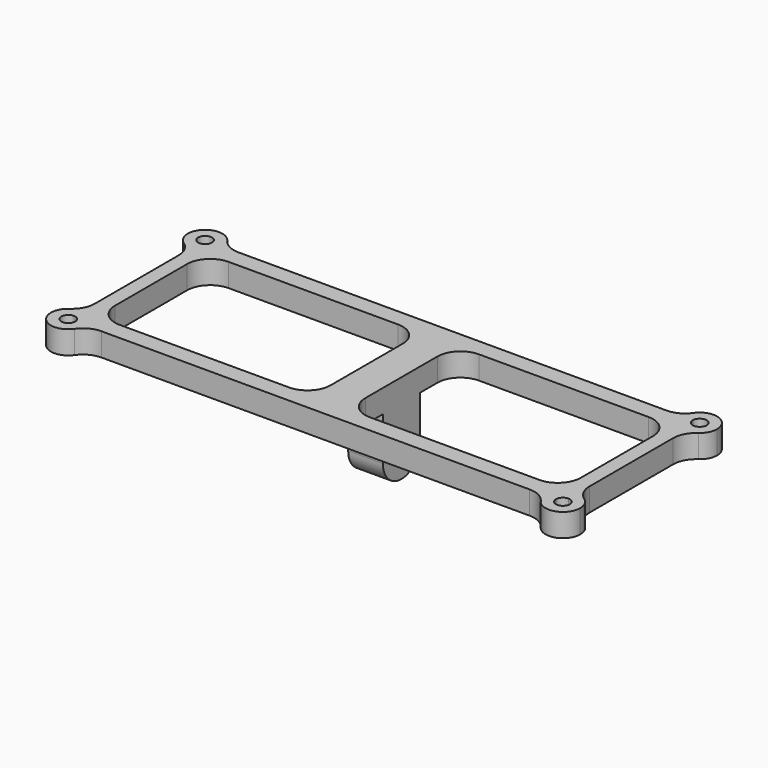
from build123d import *

# Parameters (mm, degrees)
F0_W     = 3
F0_H     = 0.7113954189
F0_H_2   = 11.7951147258
F1_DEPTH = 2
F2_R     = 2
F3_W     = 4
F3_H     = 7.7592988014
F3_R     = 0.75
F4_DEPTH = 3
F5_R     = 1.99999


# Not quite as in the source:
# - a fillet or chamfer is up to 0.001 mm smaller than in the source, because OpenCascade refuses the exact size


with BuildPart() as f1:
    # F0 (on Top) → F1 (new body)
    with BuildSketch(Plane.XY):
        with BuildLine():
            ThreePointArc((-21.4, 5.9), (-20.3393398282, 6.3393398282), (-19.9, 7.4))
            Line((-19.9, 7.4), (-20.8, 7.4))
            ThreePointArc((-20.8, 7.4), (-20.9757359313, 6.9757359313), (-21.4, 6.8))
            Line((-21.4, 6.8), (-21.4, 5.9))
        make_face()
        with BuildLine():
            Line((-20.8, 7.4), (-19.9, 7.4))
            ThreePointArc((-19.9, 7.4), (-22.4606601718, 8.4606601718), (-21.4, 5.9))
            Line((-21.4, 5.9), (-21.4, 6.8))
            ThreePointArc((-21.4, 6.8), (-21.8242640687, 7.8242640687), (-20.8, 7.4))
        make_face()
        with BuildLine():
            Line((19.9, 7.4), (-19.9, 7.4))
            ThreePointArc((-19.9, 7.4), (-20.3393398282, 6.3393398282), (-21.4, 5.9))
            Line((-21.4, 5.9), (-21.4, -5.9))
            ThreePointArc((-21.4, -5.9), (-20.3393398282, -6.3393398282), (-19.9, -7.4))
            Line((-19.9, -7.4), (19.9, -7.4))
            ThreePointArc((19.9, -7.4), (20.0395252165, -6.7682497618), (20.4321444846, -6.2540263086))
            Line((20.4321444846, -6.2540263086), (20.4321444846, 6.2540263086))
            ThreePointArc((20.4321444846, 6.2540263086), (20.0395252165, 6.7682497618), (19.9, 7.4))
        make_face()
        Polygon((-1.5, 5.8975573629), (-1.5, 6.6089527819), (1.5, 6.6089527819), (1.5, 5.8975573629), (20.1555918902, 5.8975573629), (20.1555918902, -5.8975573629), (1.5, -5.8975573629), (1.5, -6.6089527819), (-1.5, -6.6089527819), (-1.5, -5.8975573629), (-20.1555918902, -5.8975573629), (-20.1555918902, 5.8975573629), align=None, mode=Mode.SUBTRACT)
        with BuildLine():
            ThreePointArc((22.9, 7.4), (21.4, 8.9), (19.9, 7.4))
            Line((19.9, 7.4), (20.8, 7.4))
            ThreePointArc((20.8, 7.4), (21.4, 8), (22, 7.4))
            ThreePointArc((22, 7.4), (21.8242640687, 6.9757359313), (21.4, 6.8))
            Line((21.4, 6.8), (21.4, 5.9))
            ThreePointArc((21.4, 5.9), (22.4606601718, 6.3393398282), (22.9, 7.4))
        make_face()
        with BuildLine():
            Line((20.8, 7.4), (19.9, 7.4))
            ThreePointArc((19.9, 7.4), (20.0395252165, 6.7682497618), (20.4321444846, 6.2540263086))
            ThreePointArc((20.4321444846, 6.2540263086), (20.8847139324, 5.9912841775), (21.4, 5.9))
            Line((21.4, 5.9), (21.4, 6.8))
            ThreePointArc((21.4, 6.8), (20.9757359313, 6.9757359313), (20.8, 7.4))
        make_face()
        with BuildLine():
            ThreePointArc((21.4, 5.9), (20.8847139324, 5.9912841775), (20.4321444846, 6.2540263086))
            Line((20.4321444846, 6.2540263086), (20.4321444846, -6.2540263086))
            ThreePointArc((20.4321444846, -6.2540263086), (20.8847139324, -5.9912841775), (21.4, -5.9))
            Line((21.4, -5.9), (21.4, 5.9))
        make_face()
        with BuildLine():
            ThreePointArc((-19.9, -7.4), (-20.3393398282, -6.3393398282), (-21.4, -5.9))
            Line((-21.4, -5.9), (-21.4, -6.8))
            ThreePointArc((-21.4, -6.8), (-20.9757359313, -6.9757359313), (-20.8, -7.4))
            Line((-20.8, -7.4), (-19.9, -7.4))
        make_face()
        with BuildLine():
            Line((-21.4, -6.8), (-21.4, -5.9))
            ThreePointArc((-21.4, -5.9), (-22.4606601718, -8.4606601718), (-19.9, -7.4))
            Line((-19.9, -7.4), (-20.8, -7.4))
            ThreePointArc((-20.8, -7.4), (-21.8242640687, -7.8242640687), (-21.4, -6.8))
        make_face()
        with BuildLine():
            ThreePointArc((21.4, -5.9), (20.8847139324, -5.9912841775), (20.4321444846, -6.2540263086))
            ThreePointArc((20.4321444846, -6.2540263086), (20.0395252165, -6.7682497618), (19.9, -7.4))
            Line((19.9, -7.4), (20.8, -7.4))
            ThreePointArc((20.8, -7.4), (20.9757359313, -6.9757359313), (21.4, -6.8))
            Line((21.4, -6.8), (21.4, -5.9))
        make_face()
        with BuildLine():
            ThreePointArc((22.9, -7.4), (22.4606601718, -6.3393398282), (21.4, -5.9))
            Line((21.4, -5.9), (21.4, -6.8))
            ThreePointArc((21.4, -6.8), (21.8242640687, -6.9757359313), (22, -7.4))
            ThreePointArc((22, -7.4), (21.4, -8), (20.8, -7.4))
            Line((20.8, -7.4), (19.9, -7.4))
            ThreePointArc((19.9, -7.4), (21.4, -8.9), (22.9, -7.4))
        make_face()
        with Locations((0, 6.2532550724)):
            Rectangle(F0_W, F0_H)
        with Locations((0, -6.2532550724)):
            Rectangle(F0_W, F0_H)
        Rectangle(F0_W, F0_H_2)
    extrude(amount=F1_DEPTH)

    # F2
    f2_edges = [f1.edges().sort_by_distance(p)[0] for p in [
        (-19.9, 7.4, 1),
        (-19.9, -7.4, 1),
        (-1.5, -5.897557, 1),
        (-20.155592, -5.897557, 1),
        (-20.155592, 5.897557, 1),
        (20.155592, 5.897557, 1),
        (20.155592, -5.897557, 1),
        (1.5, 5.897557, 1),
        (-1.5, 5.897557, 1),
        (1.5, -5.897557, 1),
        (-21.4, 5.9, 1),
        (-21.4, -5.9, 1),
        (19.9, -7.4, 1),
        (21.4, -5.9, 1),
        (21.4, 5.9, 1),
        (19.9, 7.4, 1),
    ]]
    fillet(f2_edges, radius=F2_R)

    # F3 (on face) → F4 (join, through all)
    with BuildSketch(Plane.YZ.offset(1.5)):
        with Locations((0, -1.8796494007)):
            Rectangle(F3_W, F3_H)
        with Locations((0, -3.7315103691)):
            Circle(F3_R, mode=Mode.SUBTRACT)
    extrude(amount=-F4_DEPTH)

    # F5 (radius 2 in the source; OpenCascade refuses exactly that, so slightly less here)
    f5_edges = [f1.edges().sort_by_distance(p)[0] for p in [
        (0, 2, -5.759299),
        (0, -2, -5.759299),
    ]]
    fillet(f5_edges, radius=F5_R)


solid = f1.part
